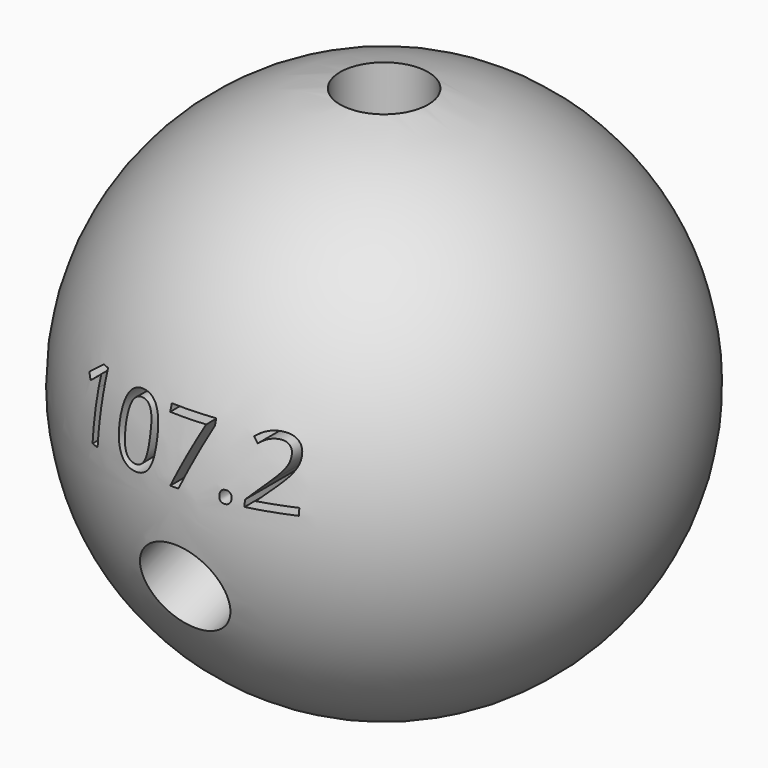
from build123d import *

# Parameters (mm, degrees)
F5_R          = 3.175
F6_DEPTH      = 50.8
F7_ANGLE      = 107.2
F10_TEXT_SIZE = 6.5466334086
F11_DEPTH     = 6.35


# Not quite as in the source:
# - Text() gives the source's letters only with a copy of the font that has no kerning and outlines rounded to 1/6400 em; it was checked with that copy


with BuildPart() as f2:
    # F1 (on Top) → F2 (revolve)
    with BuildSketch(Plane.XY):
        with BuildLine():
            Line((0, -19.05), (0, 19.05))
            ThreePointArc((0, 19.05), (-19.05, 0), (0, -19.05))
        make_face()
    revolve(axis=Axis((0, 0, 0), (0, -1, 0)))


with BuildPart() as f6:
    # F5 (on offset) → F6 (new body)
    with BuildSketch(Plane.XY.offset(7.62)):
        Circle(F5_R)
    extrude(amount=F6_DEPTH)


with BuildPart() as f7_1:
    # F7: copy of F6
    add(f6.part.rotate(Axis((38.6223383248, 0, 0), (1, 0, 0)), F7_ANGLE))


with BuildPart() as f2_1:
    add(f2.part)

    # F8: cut F6, F7_1
    add(f6.part, mode=Mode.SUBTRACT)
    add(f7_1.part, mode=Mode.SUBTRACT)

    # F10 (on offset) → F11 (cut)
    with BuildSketch(Plane.XZ.offset(19.05)):
        with Locations((-8.6203315295, 1.1972638313)):
            Text('107.2', F10_TEXT_SIZE, font='Open Sans', text_align=(TextAlign.LEFT, TextAlign.BOTTOM))
    extrude(amount=-F11_DEPTH, mode=Mode.SUBTRACT)


solid = f2_1.part
